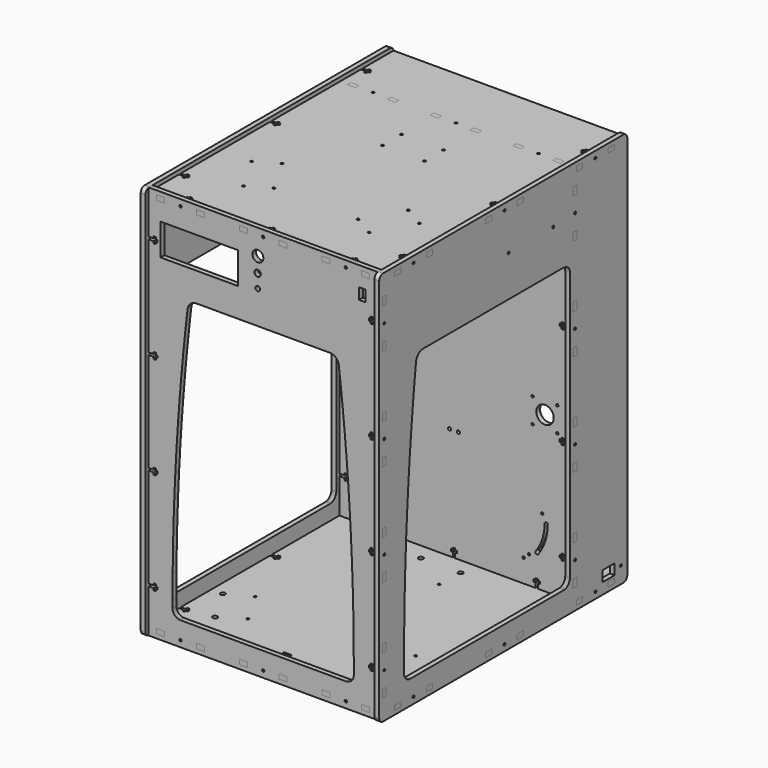
from build123d import *

# Parameters (mm, degrees)
F2_R      = 1.5
F2_W      = 10
F2_H      = 6
F3_DEPTH  = 6
F4_R      = 3
F4_R_2    = 1.5
F4_W      = 10
F4_H      = 6
F4_H_2    = 6.01
F4_W_2    = 5
F4_H_3    = 5
F5_DEPTH  = 6
F8_W      = 6
F8_H      = 10
F8_W_2    = 10
F8_H_2    = 6
F8_R      = 1.5
F8_W_3    = 19
F8_H_3    = 13.3
F9_DEPTH  = 6
F10_R     = 1.5
F11_DEPTH = 6
F13_W     = 10
F13_H     = 6
F13_W_2   = 97.175341
F13_H_2   = 39.69992
F14_DEPTH = 6
F16_R     = 1.5
F16_R_2   = 11
F16_R_3   = 2
F16_W     = 12
F16_H     = 30
F17_DEPTH = 6


# Not quite as in the source:
# - ends of sketch curves that miss each other by under 0.0002 mm in the source are joined


with BuildPart() as f3:
    # F2 (on offset) → F3 (new body)
    with BuildSketch(Plane.XY.offset(237.15)):
        Polygon((-150, 159.5), (-144, 159.5), (-144, 141), (-138, 141), (-138, 143.5), (-135, 143.5), (-135, 141), (-133, 141), (-133, 138), (-135, 138), (-135, 135.5), (-138, 135.5), (-138, 138), (-144, 138), (-144, 119.5), (-150, 119.5), (-150, 109.5), (-144, 109.5), (-144, 26.50564), (-150, 26.50564), (-150, 16.50564), (-144, 16.50564), (-144, -1.99436), (-138, -1.99436), (-138, 0.50564), (-135, 0.50564), (-135, -1.99436), (-133, -1.99436), (-133, -4.99436), (-135, -4.99436), (-135, -7.49436), (-138, -7.49436), (-138, -4.99436), (-144, -4.99436), (-144, -23.49436), (-150, -23.49436), (-150, -33.49436), (-144, -33.49436), (-144, -116.493928), (-150, -116.493928), (-150, -126.493928), (-144, -126.493928), (-144, -144.993928), (-138, -144.993928), (-138, -142.493928), (-135, -142.493928), (-135, -144.993928), (-133, -144.993928), (-133, -147.993928), (-135, -147.993928), (-135, -150.493928), (-138, -150.493928), (-138, -147.993928), (-144, -147.993928), (-144, -166.493928), (-150, -166.493928), (-150, -176.493928), (-144, -176.493928), (-144, -189.5), (-134, -189.500001), (-134, -195.500018), (-124, -195.500018), (-124, -189.500001), (-105.5, -189.500001), (-105.5, -183.5), (-108, -183.5), (-108, -180.500001), (-105.5, -180.500001), (-105.5, -178.5), (-102.5, -178.5), (-102.5, -180.500001), (-100, -180.500001), (-100, -183.5), (-102.5, -183.5), (-102.5, -189.500001), (-84, -189.500001), (-84, -195.500018), (-74, -195.500018), (-74, -189.500001), (-30, -189.5), (-30, -195.500018), (-20, -195.500018), (-20, -189.5), (-1.5, -189.5), (-1.5, -183.5), (-4, -183.5), (-4, -180.5), (-1.5, -180.5), (-1.5, -178.5), (1.5, -178.5), (1.5, -180.5), (4, -180.5), (4, -183.5), (1.5, -183.5), (1.5, -189.5), (20, -189.5), (20, -195.500018), (30, -195.500018), (30, -189.5), (74, -189.5), (74, -195.500018), (84, -195.500018), (84, -189.5), (102.5, -189.5), (102.5, -183.5), (100, -183.5), (100, -180.5), (102.5, -180.5), (102.5, -178.5), (105.5, -178.5), (105.5, -180.5), (108, -180.5), (108, -183.5), (105.5, -183.5), (105.5, -189.5), (124, -189.5), (124, -195.500018), (134, -195.500018), (134, -189.5), (144, -189.500001), (144, -176.49978), (150, -176.49978), (150, -166.49978), (144, -166.49978), (144, -147.99978), (138, -147.99978), (138, -150.49978), (135, -150.49978), (135, -147.99978), (133, -147.99978), (133, -144.99978), (135, -144.99978), (135, -142.49978), (138, -142.49978), (138, -144.99978), (144, -144.99978), (144, -126.49978), (150, -126.49978), (150, -116.49978), (144, -116.49978), (144, -33.500211), (150, -33.500211), (150, -23.500211), (144, -23.500211), (144, -5.000211), (138, -5.000211), (138, -7.500211), (135, -7.500211), (135, -5.000211), (133, -5.000211), (133, -2.000211), (135, -2.000211), (135, 0.499789), (138, 0.499789), (138, -2.000211), (144, -2.000211), (144, 16.499789), (150, 16.499789), (150, 26.499789), (144, 26.499789), (144, 109.494148), (150, 109.494148), (150, 119.494148), (144, 119.494148), (144, 137.994148), (138, 137.994148), (138, 135.494148), (135, 135.494148), (135, 137.994148), (133, 137.994148), (133, 140.994148), (135, 140.994148), (135, 143.494148), (138, 143.494148), (138, 140.994148), (144, 140.994148), (144, 159.494148), (150, 159.494148), (150, 169.494148), (144, 169.494148), (144, 189.5), (-144, 189.5), (-144, 169.5), (-150, 169.5), align=None)
        with Locations((-78.981705, -127.549038)):
            Circle(F2_R, mode=Mode.SUBTRACT)
        with Locations((-53.000943, -112.549038)):
            Circle(F2_R, mode=Mode.SUBTRACT)
        with Locations((-105.481705, -81.649692)):
            Circle(F2_R, mode=Mode.SUBTRACT)
        with Locations((-79.500943, -66.649692)):
            Circle(F2_R, mode=Mode.SUBTRACT)
        with Locations((53.000943, -112.549038)):
            Circle(F2_R, mode=Mode.SUBTRACT)
        with Locations((78.981706, -127.549038)):
            Circle(F2_R, mode=Mode.SUBTRACT)
        with Locations((105.481706, -81.649692)):
            Circle(F2_R, mode=Mode.SUBTRACT)
        with Locations((79.500943, -66.649692)):
            Circle(F2_R, mode=Mode.SUBTRACT)
        with Locations((-26.5, 25.150635)):
            Circle(F2_R, mode=Mode.SUBTRACT)
        with Locations((-26.5, 55.150635)):
            Circle(F2_R, mode=Mode.SUBTRACT)
        with Locations((-129, 107.5)):
            Rectangle(F2_W, F2_H, mode=Mode.SUBTRACT)
        with Locations((-104, 107.5)):
            Circle(F2_R, mode=Mode.SUBTRACT)
        with Locations((-79, 107.5)):
            Rectangle(F2_W, F2_H, mode=Mode.SUBTRACT)
        with Locations((-25, 107.5)):
            Rectangle(F2_W, F2_H, mode=Mode.SUBTRACT)
        with Locations((26.5, 25.150635)):
            Circle(F2_R, mode=Mode.SUBTRACT)
        with Locations((26.5, 55.150635)):
            Circle(F2_R, mode=Mode.SUBTRACT)
        with Locations((0, 107.5)):
            Circle(F2_R, mode=Mode.SUBTRACT)
        with Locations((25, 107.5)):
            Rectangle(F2_W, F2_H, mode=Mode.SUBTRACT)
        with Locations((79.000003, 107.505851)):
            Rectangle(F2_W, F2_H, mode=Mode.SUBTRACT)
        with Locations((104.000003, 107.505851)):
            Circle(F2_R, mode=Mode.SUBTRACT)
        with Locations((129.000003, 107.505851)):
            Rectangle(F2_W, F2_H, mode=Mode.SUBTRACT)
    extrude(amount=F3_DEPTH)


with BuildPart() as f5:
    # F4 (on offset) → F5 (new body)
    with BuildSketch(Plane.XY.offset(-237.15)):
        Polygon((134, -195.5000055), (134, -189.5000055), (144, -189.5000055), (144, -176.4997665), (150, -176.4997665), (150, -166.4997665), (144, -166.4997665), (144, -147.9997665), (138, -147.9997665), (138, -150.4997665), (135, -150.4997665), (135, -147.9997665), (133, -147.9997665), (133, -144.9997665), (135, -144.9997665), (135, -142.4997665), (138, -142.4997665), (138, -144.9997665), (144, -144.9997665), (144, -126.4997665), (150, -126.4997665), (150, -116.4997665), (144, -116.4997665), (144, -33.5001985), (150, -33.5001985), (150, -23.5001985), (144, -23.5001985), (144, -5.0001985), (138, -5.0001985), (138, -7.5001985), (135, -7.5001985), (135, -5.0001985), (133, -5.0001985), (133, -2.0001985), (135, -2.0001985), (135, 0.4998015), (138, 0.4998015), (138, -2.0001985), (144, -2.0001985), (144, 16.4998015), (150, 16.4998015), (150, 26.4998015), (144, 26.4998015), (144, 109.5000125), (150, 109.5000125), (150, 119.5000125), (144, 119.5000125), (144, 138.0000125), (138, 138.0000125), (138, 135.5000125), (135, 135.5000125), (135, 138.0000125), (133, 138.0000125), (133, 141.0000125), (135, 141.0000125), (135, 143.5000125), (138, 143.5000125), (138, 141.0000125), (144, 141.0000125), (144, 159.5000125), (150, 159.5000125), (150, 169.5000125), (144, 169.5000125), (144, 189.5000055), (-144, 189.5000055), (-144, 169.5000065), (-150, 169.5000065), (-150, 159.5000065), (-144, 159.5000065), (-144, 141.0000065), (-138, 141.0000065), (-138, 143.5000065), (-135, 143.5000065), (-135, 141.0000065), (-133, 141.0000065), (-133, 138.0000065), (-135, 138.0000065), (-135, 135.5000065), (-138, 135.5000065), (-138, 138.0000065), (-144, 138.0000065), (-144, 119.5000065), (-150, 119.5000065), (-150, 109.5000065), (-144, 109.5000065), (-144, 26.4998015), (-150, 26.4998015), (-150, 16.4998015), (-144, 16.4998015), (-144, -2.0001985), (-138, -2.0001985), (-138, 0.4998015), (-135, 0.4998015), (-135, -2.0001985), (-133, -2.0001985), (-133, -5.0001985), (-135, -5.0001985), (-135, -7.5001985), (-138, -7.5001985), (-138, -5.0001985), (-144, -5.0001985), (-144, -23.5001985), (-150, -23.5001985), (-150, -33.5001985), (-144, -33.5001985), (-144, -116.4997665), (-150, -116.4997665), (-150, -126.4997665), (-144, -126.4997665), (-144, -144.9997665), (-138, -144.9997665), (-138, -142.4997665), (-135, -142.4997665), (-135, -144.9997665), (-133, -144.9997665), (-133, -147.9997665), (-135, -147.9997665), (-135, -150.4997665), (-138, -150.4997665), (-138, -147.9997665), (-144, -147.9997665), (-144, -166.4997665), (-150, -166.4997665), (-150, -176.4997665), (-144, -176.4997665), (-144, -189.5000055), (-134, -189.5000055), (-134, -195.5000055), (-124, -195.5000055), (-124, -189.5000055), (-105.5, -189.5000055), (-105.5, -183.5000055), (-108, -183.5000055), (-108, -180.5000055), (-105.5, -180.5000055), (-105.5, -178.5000055), (-102.5, -178.5000055), (-102.5, -180.5000055), (-100, -180.5000055), (-100, -183.5000055), (-102.5, -183.5000055), (-102.5, -189.5000055), (-84, -189.5000055), (-84, -195.5000055), (-74, -195.5000055), (-74, -189.5000055), (-30, -189.5000055), (-30, -195.5000055), (-20, -195.5000055), (-20, -189.5000055), (-1.5, -189.5000055), (-1.5, -183.5000055), (-4, -183.5000055), (-4, -180.5000055), (-1.5, -180.5000055), (-1.5, -178.5000055), (1.5, -178.5000055), (1.5, -180.5000055), (4, -180.5000055), (4, -183.5000055), (1.5, -183.5000055), (1.5, -189.5000055), (20, -189.5000055), (20, -195.5000055), (30, -195.5000055), (30, -189.5000055), (74, -189.5000055), (74, -195.5000055), (84, -195.5000055), (84, -189.5000055), (102.5, -189.5000055), (102.5, -183.5000055), (100, -183.5000055), (100, -180.5000055), (102.5, -180.5000055), (102.5, -178.5000055), (105.5, -178.5000055), (105.5, -180.5000055), (108, -180.5000055), (108, -183.5000055), (105.5, -183.5000055), (105.5, -189.5000055), (124, -189.5000055), (124, -195.5000055), align=None)
        with Locations((-104.41343, -140.5001355)):
            Circle(F4_R, mode=Mode.SUBTRACT)
        with Locations((-76.946027, -123.4871225)):
            Circle(F4_R_2, mode=Mode.SUBTRACT)
        with BuildLine():
            ThreePointArc((-3.529365, -159.5495045), (-5.029365, -158.0495045), (-3.529365, -156.5495045))
            Line((-3.529365, -156.5495045), (3.470635, -156.5495045))
            ThreePointArc((3.470635, -156.5495045), (4.970635, -158.0495045), (3.470635, -159.5495045))
            Line((3.470635, -159.5495045), (-3.529365, -159.5495045))
        make_face(mode=Mode.SUBTRACT)
        with Locations((-129.41343, -97.1988655)):
            Circle(F4_R, mode=Mode.SUBTRACT)
        with Locations((-100.946027, -81.9179035)):
            Circle(F4_R_2, mode=Mode.SUBTRACT)
        with Locations((76.946027, -123.4871225)):
            Circle(F4_R_2, mode=Mode.SUBTRACT)
        with Locations((104.41343, -140.5001355)):
            Circle(F4_R, mode=Mode.SUBTRACT)
        with Locations((100.946027, -81.9179035)):
            Circle(F4_R_2, mode=Mode.SUBTRACT)
        with Locations((129.41343, -97.1988655)):
            Circle(F4_R, mode=Mode.SUBTRACT)
        with Locations((-24, 51.3565255)):
            Circle(F4_R_2, mode=Mode.SUBTRACT)
        with Locations((-25, 83.6504995)):
            Circle(F4_R, mode=Mode.SUBTRACT)
        with Locations((-129, 107.4998645)):
            Rectangle(F4_W, F4_H, mode=Mode.SUBTRACT)
        with Locations((-104, 107.4998645)):
            Circle(F4_R_2, mode=Mode.SUBTRACT)
        with Locations((-79, 107.4998645)):
            Rectangle(F4_W, F4_H, mode=Mode.SUBTRACT)
        with Locations((-25, 107.4998645)):
            Rectangle(F4_W, F4_H, mode=Mode.SUBTRACT)
        with Locations((24, 51.3565255)):
            Circle(F4_R_2, mode=Mode.SUBTRACT)
        with Locations((25, 83.6504995)):
            Circle(F4_R, mode=Mode.SUBTRACT)
        with Locations((0, 107.4998645)):
            Circle(F4_R_2, mode=Mode.SUBTRACT)
        with Locations((25, 107.4998645)):
            Rectangle(F4_W, F4_H, mode=Mode.SUBTRACT)
        with Locations((79, 107.4998645)):
            Rectangle(F4_W, F4_H, mode=Mode.SUBTRACT)
        with Locations((104, 107.4998645)):
            Circle(F4_R_2, mode=Mode.SUBTRACT)
        with Locations((129, 107.5048645)):
            Rectangle(F4_W, F4_H_2, mode=Mode.SUBTRACT)
        with Locations((136.5, 117.9998645)):
            Rectangle(F4_W_2, F4_H_3, mode=Mode.SUBTRACT)
    extrude(amount=-F5_DEPTH)


with BuildPart() as f9:
    # F8 (on offset) → F9 (new body)
    with BuildSketch(Plane.YZ.offset(144)):
        with BuildLine():
            Line((189.499992, -242.15), (189.499402, 242.149892))
            Line((189.499402, 242.149892), (189.294966, 243.702831))
            Line((189.294966, 243.702831), (188.695564, 245.149942))
            Line((188.695564, 245.149942), (187.742044, 246.392606))
            Line((187.742044, 246.392606), (186.499388, 247.346136))
            Line((186.499388, 247.346136), (185.052282, 247.945551))
            Line((185.052282, 247.945551), (183.499344, 248.15))
            Line((183.499344, 248.15), (-194.499763, 248.15))
            ThreePointArc((-194.499763, 248.15), (-198.7423994455, 246.3927505531), (-200.499779, 242.150168))
            Line((-200.499779, 242.150168), (-200.499888, -242.15))
            Line((-200.499888, -242.15), (-200.295444, -243.702914))
            Line((-200.295444, -243.702914), (-199.696041, -245.15))
            Line((-199.696041, -245.15), (-198.74253, -246.392641))
            Line((-198.74253, -246.392641), (-197.499889, -247.346152))
            Line((-197.499889, -247.346152), (-196.052804, -247.945555))
            Line((-196.052804, -247.945555), (-194.49989, -248.15))
            Line((-194.49989, -248.15), (183.5, -248.15))
            ThreePointArc((183.5, -248.15), (187.7426382122, -246.3926402625), (189.499992, -242.15))
        make_face()
        with Locations((-192.500018, -217.15)):
            Rectangle(F8_W, F8_H, mode=Mode.SUBTRACT)
        with Locations((-171.49978, -240.15)):
            Rectangle(F8_W_2, F8_H_2, mode=Mode.SUBTRACT)
        with Locations((-192.500018, -192.15)):
            Circle(F8_R, mode=Mode.SUBTRACT)
        Polygon((-144.99978, -240.15), (-145.050891, -240.538229), (-145.200742, -240.9), (-145.43912, -241.21066), (-145.74978, -241.449038), (-146.111552, -241.598889), (-146.49978, -241.65), (-146.888009, -241.598889), (-147.24978, -241.449038), (-147.56044, -241.21066), (-147.798818, -240.9), (-147.948669, -240.538229), (-147.99978, -240.15), (-147.948669, -239.761771), (-147.798818, -239.4), (-147.56044, -239.08934), (-147.24978, -238.850962), (-146.888009, -238.701111), (-146.49978, -238.65), (-146.111552, -238.701111), (-145.74978, -238.850962), (-145.43912, -239.08934), (-145.200742, -239.4), (-145.050891, -239.761771), align=None, mode=Mode.SUBTRACT)
        with Locations((-121.49978, -240.15)):
            Rectangle(F8_W_2, F8_H_2, mode=Mode.SUBTRACT)
        with Locations((-192.500018, -167.15)):
            Rectangle(F8_W, F8_H, mode=Mode.SUBTRACT)
        with Locations((-28.500211, -240.15)):
            Rectangle(F8_W_2, F8_H_2, mode=Mode.SUBTRACT)
        with Locations((-192.500018, -89.05)):
            Rectangle(F8_W, F8_H, mode=Mode.SUBTRACT)
        Polygon((-191.05113, -63.661771), (-191.000018, -64.05), (-191.05113, -64.438229), (-191.20098, -64.8), (-191.439358, -65.11066), (-191.750018, -65.349038), (-192.11179, -65.498889), (-192.500018, -65.55), (-192.888247, -65.498889), (-193.250018, -65.349038), (-193.560679, -65.11066), (-193.799056, -64.8), (-193.948907, -64.438229), (-194.000018, -64.05), (-193.948907, -63.661771), (-193.799056, -63.3), (-193.560679, -62.98934), (-193.250018, -62.750962), (-192.888247, -62.601111), (-192.500018, -62.55), (-192.11179, -62.601111), (-191.750018, -62.750962), (-191.439358, -62.98934), (-191.20098, -63.3), align=None, mode=Mode.SUBTRACT)
        with Locations((-192.500018, -39.05)):
            Rectangle(F8_W, F8_H, mode=Mode.SUBTRACT)
        with BuildLine():
            Line((90.805261, -218.064449), (89.5, -218.15))
            Line((89.5, -218.15), (-151.499902, -218.15))
            Line((-151.499902, -218.15), (-152.805163, -218.064449))
            Line((-152.805163, -218.064449), (-154.088092, -217.809258))
            Line((-154.088092, -217.809258), (-155.326736, -217.388795))
            Line((-155.326736, -217.388795), (-156.499902, -216.810254))
            Line((-156.499902, -216.810254), (-157.587516, -216.083533))
            Line((-157.587516, -216.083533), (-158.570969, -215.221068))
            Line((-158.570969, -215.221068), (-159.433435, -214.237614))
            Line((-159.433435, -214.237614), (-160.160156, -213.15))
            Line((-160.160156, -213.15), (-160.738697, -211.976834))
            Line((-160.738697, -211.976834), (-161.15916, -210.73819))
            Line((-161.15916, -210.73819), (-161.41435, -209.455262))
            Line((-161.41435, -209.455262), (-161.499902, -208.15))
            Line((-161.499902, -208.15), (-161.499904, -198.15))
            Line((-161.499904, -198.15), (-161.360861, -169.976288))
            Line((-161.360861, -169.976288), (-160.943732, -141.805321))
            Line((-160.943732, -141.805321), (-160.248556, -113.639844))
            Line((-160.248556, -113.639844), (-159.275401, -85.482601))
            Line((-159.275401, -85.482601), (-158.024363, -57.336335))
            Line((-158.024363, -57.336335), (-156.495562, -29.203789))
            Line((-156.495562, -29.203789), (-154.689149, -1.087704))
            Line((-154.689149, -1.087704), (-152.605299, 27.00918))
            Line((-152.605299, 27.00918), (-150.244215, 55.084128))
            Line((-150.244215, 55.084128), (-147.606127, 83.134401))
            Line((-147.606127, 83.134401), (-144.691292, 111.157269))
            Line((-144.691292, 111.157269), (-142.64004, 129.15))
            Line((-142.64004, 129.15), (-142.402772, 130.497965))
            Line((-142.402772, 130.497965), (-142.003956, 131.80726))
            Line((-142.003956, 131.80726), (-141.449468, 133.058599))
            Line((-141.449468, 133.058599), (-140.747473, 134.23355))
            Line((-140.747473, 134.23355), (-139.908313, 135.314807))
            Line((-139.908313, 135.314807), (-138.944347, 136.286443))
            Line((-138.944347, 136.286443), (-137.869775, 137.134146))
            Line((-137.869775, 137.134146), (-136.700425, 137.845431))
            Line((-136.700425, 137.845431), (-135.45352, 138.40982))
            Line((-135.45352, 138.40982), (-134.147427, 138.819))
            Line((-134.147427, 138.819), (-132.801385, 139.066944))
            Line((-132.801385, 139.066944), (-131.435219, 139.15))
            Line((-131.435219, 139.15), (89.5, 139.15))
            ThreePointArc((89.5, 139.15), (96.5710678119, 136.2210678119), (99.5, 129.15))
            Line((99.5, 129.15), (99.5, -208.15))
            Line((99.5, -208.15), (99.414448, -209.455262))
            Line((99.414448, -209.455262), (99.159258, -210.73819))
            Line((99.159258, -210.73819), (98.738795, -211.976834))
            Line((98.738795, -211.976834), (98.160254, -213.15))
            Line((98.160254, -213.15), (97.433533, -214.237614))
            Line((97.433533, -214.237614), (96.571067, -215.221068))
            Line((96.571067, -215.221068), (95.587614, -216.083533))
            Line((95.587614, -216.083533), (94.5, -216.810254))
            Line((94.5, -216.810254), (93.326834, -217.388795))
            Line((93.326834, -217.388795), (92.08819, -217.809258))
            Line((92.08819, -217.809258), (90.805261, -218.064449))
        make_face(mode=Mode.SUBTRACT)
        Polygon((-2.439551, -239.08934), (-2.201173, -239.4), (-2.051323, -239.761771), (-2.000211, -240.15), (-2.051323, -240.538229), (-2.201173, -240.9), (-2.439551, -241.21066), (-2.750211, -241.449038), (-3.111983, -241.598889), (-3.500211, -241.65), (-3.88844, -241.598889), (-4.250211, -241.449038), (-4.560872, -241.21066), (-4.799249, -240.9), (-4.9491, -240.538229), (-5.000211, -240.15), (-4.9491, -239.761771), (-4.799249, -239.4), (-4.560872, -239.08934), (-4.250211, -238.850962), (-3.88844, -238.701111), (-3.500211, -238.65), (-3.111983, -238.701111), (-2.750211, -238.850962), align=None, mode=Mode.SUBTRACT)
        with Locations((21.499789, -240.15)):
            Rectangle(F8_W_2, F8_H_2, mode=Mode.SUBTRACT)
        with Locations((114.5, -240.15)):
            Rectangle(F8_W_2, F8_H_2, mode=Mode.SUBTRACT)
        with Locations((107.505851, -217.15)):
            Rectangle(F8_W, F8_H, mode=Mode.SUBTRACT)
        Polygon((140.56066, -239.08934), (140.799038, -239.4), (140.948888, -239.761771), (141, -240.15), (140.948888, -240.538229), (140.799038, -240.9), (140.56066, -241.21066), (140.25, -241.449038), (139.888228, -241.598889), (139.5, -241.65), (139.111771, -241.598889), (138.75, -241.449038), (138.439339, -241.21066), (138.200961, -240.9), (138.051111, -240.538229), (138, -240.15), (138.051111, -239.761771), (138.200961, -239.4), (138.439339, -239.08934), (138.75, -238.850962), (139.111771, -238.701111), (139.5, -238.65), (139.888228, -238.701111), (140.25, -238.850962), align=None, mode=Mode.SUBTRACT)
        Polygon((106.056963, -191.761771), (106.206813, -191.4), (106.445191, -191.08934), (106.755851, -190.850962), (107.117623, -190.701111), (107.505851, -190.65), (107.89408, -190.701111), (108.255851, -190.850962), (108.566511, -191.08934), (108.804889, -191.4), (108.95474, -191.761771), (109.005851, -192.15), (108.95474, -192.538229), (108.804889, -192.9), (108.566511, -193.21066), (108.255851, -193.449038), (107.89408, -193.598889), (107.505851, -193.65), (107.117623, -193.598889), (106.755851, -193.449038), (106.445191, -193.21066), (106.206813, -192.9), (106.056963, -192.538229), (106.005851, -192.15), align=None, mode=Mode.SUBTRACT)
        with Locations((164.5, -240.15)):
            Rectangle(F8_W_2, F8_H_2, mode=Mode.SUBTRACT)
        with Locations((160.1, -227.5)):
            Rectangle(F8_W_3, F8_H_3, mode=Mode.SUBTRACT)
        with Locations((179.500025, -227.500622)):
            Circle(F8_R, mode=Mode.SUBTRACT)
        with Locations((107.505851, -167.15)):
            Rectangle(F8_W, F8_H, mode=Mode.SUBTRACT)
        with Locations((107.505851, -89.05)):
            Rectangle(F8_W, F8_H, mode=Mode.SUBTRACT)
        Polygon((107.505851, -62.55), (107.89408, -62.601111), (108.255851, -62.750962), (108.566511, -62.98934), (108.804889, -63.3), (108.95474, -63.661771), (109.005851, -64.05), (108.95474, -64.438229), (108.804889, -64.8), (108.566511, -65.11066), (108.255851, -65.349038), (107.89408, -65.498889), (107.505851, -65.55), (107.117623, -65.498889), (106.755851, -65.349038), (106.445191, -65.11066), (106.206813, -64.8), (106.056963, -64.438229), (106.005851, -64.05), (106.056963, -63.661771), (106.206813, -63.3), (106.445191, -62.98934), (106.755851, -62.750962), (107.117623, -62.601111), align=None, mode=Mode.SUBTRACT)
        with Locations((107.505851, -39.05)):
            Rectangle(F8_W, F8_H, mode=Mode.SUBTRACT)
        with Locations((-192.500018, 39.05)):
            Rectangle(F8_W, F8_H, mode=Mode.SUBTRACT)
        Polygon((-192.11179, 62.601111), (-192.500018, 62.55), (-192.888247, 62.601111), (-193.250018, 62.750962), (-193.560679, 62.98934), (-193.799056, 63.3), (-193.948907, 63.661771), (-194.000018, 64.05), (-193.948907, 64.438229), (-193.799056, 64.8), (-193.560679, 65.11066), (-193.250018, 65.349038), (-192.888247, 65.498889), (-192.500018, 65.55), (-192.11179, 65.498889), (-191.750018, 65.349038), (-191.439358, 65.11066), (-191.20098, 64.8), (-191.05113, 64.438229), (-191.000018, 64.05), (-191.05113, 63.661771), (-191.20098, 63.3), (-191.439358, 62.98934), (-191.750018, 62.750962), align=None, mode=Mode.SUBTRACT)
        with Locations((-192.500018, 89.05)):
            Rectangle(F8_W, F8_H, mode=Mode.SUBTRACT)
        with Locations((-192.500018, 167.15)):
            Rectangle(F8_W, F8_H, mode=Mode.SUBTRACT)
        Polygon((-192.888247, 190.701111), (-193.250018, 190.850962), (-193.560679, 191.08934), (-193.799056, 191.4), (-193.948907, 191.761771), (-194.000018, 192.15), (-193.948907, 192.538229), (-193.799056, 192.9), (-193.560679, 193.21066), (-193.250018, 193.449038), (-192.888247, 193.598889), (-192.500018, 193.65), (-192.11179, 193.598889), (-191.750018, 193.449038), (-191.439358, 193.21066), (-191.20098, 192.9), (-191.05113, 192.538229), (-191.000018, 192.15), (-191.05113, 191.761771), (-191.20098, 191.4), (-191.439358, 191.08934), (-191.750018, 190.850962), (-192.11179, 190.701111), (-192.500018, 190.65), align=None, mode=Mode.SUBTRACT)
        with Locations((-192.500018, 217.15)):
            Rectangle(F8_W, F8_H, mode=Mode.SUBTRACT)
        with Locations((-171.49978, 240.15)):
            Rectangle(F8_W_2, F8_H_2, mode=Mode.SUBTRACT)
        Polygon((-145.050891, 240.538229), (-144.99978, 240.15), (-145.050891, 239.761771), (-145.200742, 239.4), (-145.43912, 239.08934), (-145.74978, 238.850962), (-146.111552, 238.701111), (-146.49978, 238.65), (-146.888009, 238.701111), (-147.24978, 238.850962), (-147.56044, 239.08934), (-147.798818, 239.4), (-147.948669, 239.761771), (-147.99978, 240.15), (-147.948669, 240.538229), (-147.798818, 240.9), (-147.56044, 241.21066), (-147.24978, 241.449038), (-146.888009, 241.598889), (-146.49978, 241.65), (-146.111552, 241.598889), (-145.74978, 241.449038), (-145.43912, 241.21066), (-145.200742, 240.9), align=None, mode=Mode.SUBTRACT)
        with Locations((-121.49978, 240.15)):
            Rectangle(F8_W_2, F8_H_2, mode=Mode.SUBTRACT)
        with Locations((-28.500211, 240.15)):
            Rectangle(F8_W_2, F8_H_2, mode=Mode.SUBTRACT)
        with Locations((107.505851, 39.05)):
            Rectangle(F8_W, F8_H, mode=Mode.SUBTRACT)
        with Locations((107.505851, 64.05)):
            Circle(F8_R, mode=Mode.SUBTRACT)
        with Locations((107.505851, 89.05)):
            Rectangle(F8_W, F8_H, mode=Mode.SUBTRACT)
        with Locations((3.031226, 190.6)):
            Circle(F8_R, mode=Mode.SUBTRACT)
        Polygon((-2.051323, 239.761771), (-2.201173, 239.4), (-2.439551, 239.08934), (-2.750211, 238.850962), (-3.111983, 238.701111), (-3.500211, 238.65), (-3.88844, 238.701111), (-4.250211, 238.850962), (-4.560872, 239.08934), (-4.799249, 239.4), (-4.9491, 239.761771), (-5.000211, 240.15), (-4.9491, 240.538229), (-4.799249, 240.9), (-4.560872, 241.21066), (-4.250211, 241.449038), (-3.88844, 241.598889), (-3.500211, 241.65), (-3.111983, 241.598889), (-2.750211, 241.449038), (-2.439551, 241.21066), (-2.201173, 240.9), (-2.051323, 240.538229), (-2.000211, 240.15), align=None, mode=Mode.SUBTRACT)
        with Locations((21.499789, 240.15)):
            Rectangle(F8_W_2, F8_H_2, mode=Mode.SUBTRACT)
        Polygon((71.582337, 190.988229), (71.732188, 191.35), (71.970566, 191.66066), (72.281226, 191.899038), (72.642998, 192.048889), (73.031226, 192.1), (73.419455, 192.048889), (73.781226, 191.899038), (74.091886, 191.66066), (74.330264, 191.35), (74.480115, 190.988229), (74.531226, 190.6), (74.480115, 190.211771), (74.330264, 189.85), (74.091886, 189.53934), (73.781226, 189.300962), (73.419455, 189.151111), (73.031226, 189.1), (72.642998, 189.151111), (72.281226, 189.300962), (71.970566, 189.53934), (71.732188, 189.85), (71.582337, 190.211771), (71.531226, 190.6), align=None, mode=Mode.SUBTRACT)
        with Locations((107.5, 167.15)):
            Rectangle(F8_W, F8_H, mode=Mode.SUBTRACT)
        Polygon((106.200961, 192.9), (106.439339, 193.21066), (106.75, 193.449038), (107.111771, 193.598889), (107.5, 193.65), (107.888228, 193.598889), (108.25, 193.449038), (108.56066, 193.21066), (108.799038, 192.9), (108.948888, 192.538229), (109, 192.15), (108.948888, 191.761771), (108.799038, 191.4), (108.56066, 191.08934), (108.25, 190.850962), (107.888228, 190.701111), (107.5, 190.65), (107.111771, 190.701111), (106.75, 190.850962), (106.439339, 191.08934), (106.200961, 191.4), (106.051111, 191.761771), (106, 192.15), (106.051111, 192.538229), align=None, mode=Mode.SUBTRACT)
        with Locations((107.5, 217.15)):
            Rectangle(F8_W, F8_H, mode=Mode.SUBTRACT)
        with Locations((114.494148, 240.15)):
            Rectangle(F8_W_2, F8_H_2, mode=Mode.SUBTRACT)
        Polygon((139.105919, 241.598889), (139.494148, 241.65), (139.882376, 241.598889), (140.244148, 241.449038), (140.554808, 241.21066), (140.793186, 240.9), (140.943037, 240.538229), (140.994148, 240.15), (140.943037, 239.761771), (140.793186, 239.4), (140.554808, 239.08934), (140.244148, 238.850962), (139.882376, 238.701111), (139.494148, 238.65), (139.105919, 238.701111), (138.744148, 238.850962), (138.433488, 239.08934), (138.19511, 239.4), (138.045259, 239.761771), (137.994148, 240.15), (138.045259, 240.538229), (138.19511, 240.9), (138.433488, 241.21066), (138.744148, 241.449038), align=None, mode=Mode.SUBTRACT)
        with Locations((164.494148, 240.15)):
            Rectangle(F8_W_2, F8_H_2, mode=Mode.SUBTRACT)
    extrude(amount=F9_DEPTH)


with BuildPart() as f11:
    # F10 (on offset) → F11 (new body)
    with BuildSketch(Plane(origin=(-144, 0, 0), x_dir=(0, -1, 0), z_dir=(-1, 0, 0))):
        with BuildLine():
            Line((-189.4994047464, 242.1501386605), (-189.5003987455, -242.1498613388))
            Line((-189.5003987455, -242.1498613388), (-189.2959570666, -243.7027755127))
            Line((-189.2959570666, -243.7027755127), (-188.6965572976, -245.1498610227))
            Line((-188.6965572976, -245.1498610227), (-187.7430483547, -246.3925028338))
            Line((-187.7430483547, -246.3925028338), (-186.5004091659, -247.3460158909))
            Line((-186.5004091659, -247.3460158909), (-185.0533246758, -247.945420122))
            Line((-185.0533246758, -247.945420122), (-183.5004118497, -248.1498664431))
            Line((-183.5004118497, -248.1498664431), (194.5006771501, -248.1501880126))
            ThreePointArc((194.5006771501, -248.1501880126), (198.7425492927, -246.393151269), (200.4995932535, -242.1512821159))
            Line((200.4995932535, -242.1512821159), (200.4997992534, 242.1497908841))
            ThreePointArc((200.4997992534, 242.1497908841), (198.7424291669, 246.3924452898), (194.4997733577, 248.1498119884))
            Line((194.4997733577, 248.1498119884), (-183.4993926421, 248.1501335562))
            ThreePointArc((-183.4993926421, 248.1501335562), (-187.7420372991, 246.3927782772), (-189.4994047464, 242.1501386605))
        make_face()
        Polygon((-159.5004015962, -243.1498868601), (-169.5004015962, -243.149878353), (-169.5003964919, -237.149878353), (-159.5003964919, -237.1498868601), align=None, mode=Mode.SUBTRACT)
        with Locations((-139.5003990441, -240.1499038743)):
            Circle(F10_R, mode=Mode.SUBTRACT)
        Polygon((-109.5004015962, -243.1499293957), (-119.5004015962, -243.1499208886), (-119.5003964919, -237.1499208886), (-109.500396492, -237.1499293957), align=None, mode=Mode.SUBTRACT)
        Polygon((-104.5062417313, -222.1499336442), (-110.5062417313, -222.14992854), (-110.5062332242, -212.14992854), (-104.5062332242, -212.1499336442), align=None, mode=Mode.SUBTRACT)
        with Locations((-107.50621621, -192.1499310921)):
            Circle(F10_R, mode=Mode.SUBTRACT)
        Polygon((-104.5061991958, -172.1499336443), (-110.5061991958, -172.14992854), (-110.5061906887, -162.14992854), (-104.5061906887, -162.1499336443), align=None, mode=Mode.SUBTRACT)
        Polygon((-16.506043492, -237.1500085069), (-16.5060485962, -243.1500085069), (-26.5060485962, -243.1499999998), (-26.506043492, -237.1499999998), align=None, mode=Mode.SUBTRACT)
        Polygon((2.0450656256, -240.5382532886), (1.9939539559, -240.1500242451), (2.0450662861, -239.7617952886), (2.1949165939, -239.400024416), (2.4332948582, -239.0893646188), (2.743955061, -238.8509868831), (3.1057271885, -238.7011361909), (3.4939552319, -238.6500255211), (3.8821841885, -238.7011368514), (4.243955061, -238.8509881592), (4.5546158582, -239.0893664235), (4.7929925939, -239.4000266262), (4.9428432861, -239.7617977537), (4.9939539559, -240.1500267972), (4.9428426256, -240.5382557537), (4.7929913178, -240.9000266262), (4.5546140536, -241.2106864235), (4.2439528508, -241.4490641592), (3.8821817233, -241.5989148514), (3.4939526798, -241.6500255211), (3.1057247233, -241.5989141909), (2.7439528508, -241.4490628831), (2.4332930536, -241.2106846188), (2.1949153178, -240.900024416), align=None, mode=Mode.SUBTRACT)
        Polygon((-110.5061242482, -84.04992854), (-104.5061242482, -84.0499336443), (-104.5061327553, -94.0499336443), (-110.5061327553, -94.04992854), align=None, mode=Mode.SUBTRACT)
        Polygon((-107.50610851, -65.5499310922), (-107.8943364666, -65.4988197619), (-108.2561083391, -65.3489684541), (-108.5667681363, -65.1105901898), (-108.805145872, -64.7999299871), (-108.9549955642, -64.4381588596), (-109.006107234, -64.0499298161), (-108.9549949037, -63.6617008596), (-108.8051445959, -63.2999299871), (-108.5667663317, -62.9892701898), (-108.2561061289, -62.7508924541), (-107.8943340014, -62.6010417619), (-107.5061059579, -62.5499310922), (-107.1178770014, -62.6010424224), (-106.7561061289, -62.7508937302), (-106.4454453317, -62.9892719945), (-106.2070675959, -63.2999321973), (-106.0572179037, -63.6617033247), (-106.006107234, -64.0499323682), (-106.0572185642, -64.4381613247), (-106.207068872, -64.7999321973), (-106.4454471363, -65.1105919945), (-106.7561083391, -65.3489697302), (-107.1178794666, -65.4988204224), align=None, mode=Mode.SUBTRACT)
        Polygon((-104.5060902198, -44.0499336443), (-110.5060902198, -44.04992854), (-110.5060817127, -34.04992854), (-104.5060817127, -34.0499336443), align=None, mode=Mode.SUBTRACT)
        Polygon((33.4939514037, -243.1500510425), (23.4939514037, -243.1500425354), (23.493956508, -237.1500425354), (33.493956508, -237.1500510425), align=None, mode=Mode.SUBTRACT)
        Polygon((126.493525508, -237.1501301582), (126.4935204037, -243.1501301582), (116.4935204037, -243.1501216511), (116.493525508, -237.1501216511), align=None, mode=Mode.SUBTRACT)
        with Locations((146.4935229558, -240.1501471724)):
            Circle(F10_R, mode=Mode.SUBTRACT)
        Polygon((166.4935204037, -243.1501641866), (166.4935255079, -237.1501641866), (176.4935255079, -237.1501726937), (176.4935204037, -243.1501726937), align=None, mode=Mode.SUBTRACT)
        Polygon((189.4996282686, -222.1501837581), (189.4996367757, -212.1501837581), (195.4996367757, -212.1501888624), (195.4996282686, -222.1501888624), align=None, mode=Mode.SUBTRACT)
        with Locations((192.4996537899, -192.1501863103)):
            Circle(F10_R, mode=Mode.SUBTRACT)
        Polygon((195.4996793112, -162.1501888624), (195.4996708041, -172.1501888624), (189.4996708041, -172.1501837581), (189.4996793112, -162.1501837581), align=None, mode=Mode.SUBTRACT)
        with BuildLine():
            Line((159.4333047563, -214.2375476443), (158.5708387563, -215.2210016443))
            Line((158.5708387563, -215.2210016443), (157.5873857563, -216.0834666443))
            Line((157.5873857563, -216.0834666443), (156.4997717563, -216.8101876443))
            Line((156.4997717563, -216.8101876443), (155.3266057563, -217.3887286443))
            Line((155.3266057563, -217.3887286443), (154.0879617563, -217.8091916443))
            Line((154.0879617563, -217.8091916443), (152.8050327563, -218.0643826443))
            Line((152.8050327563, -218.0643826443), (151.4997717563, -218.1499336443))
            Line((151.4997717563, -218.1499336443), (-89.5001302437, -218.1499336443))
            Line((-89.5001302437, -218.1499336443), (-90.8053912437, -218.0643826443))
            Line((-90.8053912437, -218.0643826443), (-92.0883202437, -217.8091916443))
            Line((-92.0883202437, -217.8091916443), (-93.3269642437, -217.3887286443))
            Line((-93.3269642437, -217.3887286443), (-94.5001302437, -216.8101876443))
            Line((-94.5001302437, -216.8101876443), (-95.5877442437, -216.0834666443))
            Line((-95.5877442437, -216.0834666443), (-96.5711972437, -215.2210016443))
            Line((-96.5711972437, -215.2210016443), (-97.4336632437, -214.2375476443))
            Line((-97.4336632437, -214.2375476443), (-98.1603842437, -213.1499336443))
            Line((-98.1603842437, -213.1499336443), (-98.7389252437, -211.9767676443))
            Line((-98.7389252437, -211.9767676443), (-99.1593882437, -210.7381236443))
            Line((-99.1593882437, -210.7381236443), (-99.4145782437, -209.4551956443))
            Line((-99.4145782437, -209.4551956443), (-99.5001302437, -208.1499336443))
            Line((-99.5001302437, -208.1499336443), (-99.5001302437, 129.1500663557))
            ThreePointArc((-99.5001302437, 129.1500663557), (-96.5711980556, 136.2211341675), (-89.5001302437, 139.1500663557))
            Line((-89.5001302437, 139.1500663557), (131.4350887563, 139.1500663557))
            Line((131.4350887563, 139.1500663557), (132.8012547563, 139.0670103557))
            Line((132.8012547563, 139.0670103557), (134.1472967563, 138.8190663557))
            Line((134.1472967563, 138.8190663557), (135.4533897563, 138.4098863557))
            Line((135.4533897563, 138.4098863557), (136.7002947563, 137.8454973557))
            Line((136.7002947563, 137.8454973557), (137.8696447563, 137.1342123557))
            Line((137.8696447563, 137.1342123557), (138.9442167563, 136.2865093557))
            Line((138.9442167563, 136.2865093557), (139.9081827563, 135.3148733557))
            Line((139.9081827563, 135.3148733557), (140.7473427563, 134.2336163557))
            Line((140.7473427563, 134.2336163557), (141.4493377563, 133.0586653557))
            Line((141.4493377563, 133.0586653557), (142.0038257563, 131.8073263557))
            Line((142.0038257563, 131.8073263557), (142.4026417563, 130.4980313557))
            Line((142.4026417563, 130.4980313557), (142.6399097563, 129.1500663557))
            Line((142.6399097563, 129.1500663557), (144.6911617563, 111.1573353557))
            Line((144.6911617563, 111.1573353557), (147.6059967563, 83.1344673557))
            Line((147.6059967563, 83.1344673557), (150.2440847563, 55.0841943557))
            Line((150.2440847563, 55.0841943557), (152.6051687563, 27.0092463557))
            Line((152.6051687563, 27.0092463557), (154.6890187563, -1.0876376443))
            Line((154.6890187563, -1.0876376443), (156.4954317563, -29.2037226443))
            Line((156.4954317563, -29.2037226443), (158.0242327563, -57.3362686443))
            Line((158.0242327563, -57.3362686443), (159.2752707563, -85.4825346443))
            Line((159.2752707563, -85.4825346443), (160.2484257563, -113.6397776443))
            Line((160.2484257563, -113.6397776443), (160.9436017563, -141.8052546443))
            Line((160.9436017563, -141.8052546443), (161.3607307563, -169.9762216443))
            Line((161.3607307563, -169.9762216443), (161.4997737563, -198.1499336443))
            Line((161.4997737563, -198.1499336443), (161.4997717563, -208.1499336443))
            Line((161.4997717563, -208.1499336443), (161.4142197563, -209.4551956443))
            Line((161.4142197563, -209.4551956443), (161.1590297563, -210.7381236443))
            Line((161.1590297563, -210.7381236443), (160.7385667563, -211.9767676443))
            Line((160.7385667563, -211.9767676443), (160.1600257563, -213.1499336443))
            Line((160.1600257563, -213.1499336443), (159.4333047563, -214.2375476443))
        make_face(mode=Mode.SUBTRACT)
        Polygon((189.4997457517, -84.0501837582), (195.4997457517, -84.0501888624), (195.4997372446, -94.0501888624), (189.4997372446, -94.0501837582), align=None, mode=Mode.SUBTRACT)
        with Locations((192.4997627659, -64.0501863103)):
            Circle(F10_R, mode=Mode.SUBTRACT)
        Polygon((189.4997882872, -34.0501837582), (195.4997882872, -34.0501888624), (195.4997797801, -44.0501888624), (189.4997797801, -44.0501837582), align=None, mode=Mode.SUBTRACT)
        Polygon((-110.5060152722, 44.0500714599), (-104.5060152722, 44.0500663557), (-104.5060237793, 34.0500663557), (-110.5060237793, 34.0500714599), align=None, mode=Mode.SUBTRACT)
        Polygon((-106.206959896, 63.3000678027), (-106.4453381603, 62.9894080055), (-106.7559993631, 62.7510302698), (-107.1177704905, 62.6011795775), (-107.505999534, 62.5500689078), (-107.8942274905, 62.6011802381), (-108.2559993631, 62.7510315458), (-108.5666591603, 62.9894098101), (-108.805036896, 63.3000700129), (-108.9548865882, 63.6618411404), (-109.005998258, 64.0500701839), (-108.9548859277, 64.4382991404), (-108.8050356199, 64.8000700129), (-108.5666573556, 65.1107298101), (-108.2559971528, 65.3491075458), (-107.8942250254, 65.4989582381), (-107.5059969819, 65.5500689078), (-107.1177680254, 65.4989575775), (-106.7559971529, 65.3491062698), (-106.4453363556, 65.1107280055), (-106.2069586199, 64.8000678027), (-106.0571089277, 64.4382966752), (-106.005998258, 64.0500676317), (-106.0571095882, 63.6618386752), align=None, mode=Mode.SUBTRACT)
        Polygon((-104.5059812437, 84.0500663557), (-110.5059812437, 84.0500714599), (-110.5059727366, 94.0500714599), (-104.5059727366, 94.0500663556), align=None, mode=Mode.SUBTRACT)
        Polygon((-104.5000628033, 162.1500663506), (-110.5000628033, 162.1500714549), (-110.5000542962, 172.1500714549), (-104.5000542962, 172.1500663506), align=None, mode=Mode.SUBTRACT)
        Polygon((-159.4999938957, 243.1501131397), (-159.499999, 237.1501131397), (-169.499999, 237.1501216468), (-169.4999938957, 243.1501216468), align=None, mode=Mode.SUBTRACT)
        with Locations((-107.5000372819, 192.1500689028)):
            Circle(F10_R, mode=Mode.SUBTRACT)
        Polygon((-139.4999977239, 238.6500961255), (-139.8882256804, 238.7012074558), (-140.2499975529, 238.8510587635), (-140.5606573501, 239.0894370278), (-140.7990350859, 239.4000972306), (-140.9488857781, 239.7618683581), (-140.9999964478, 240.1500974016), (-140.9488851176, 240.5383263581), (-140.7990338098, 240.9000972306), (-140.5606555455, 241.2107570278), (-140.2499953427, 241.4491347635), (-139.8882232152, 241.5989854558), (-139.4999951718, 241.6500961255), (-139.1117662152, 241.5989847952), (-138.7499953427, 241.4491334875), (-138.4393355455, 241.2107552232), (-138.2009578098, 240.9000950204), (-138.0511071176, 240.5383238929), (-137.9999964478, 240.1500948494), (-138.0511077781, 239.7618658929), (-138.2009590859, 239.4000950204), (-138.4393373501, 239.0894352232), (-138.7499975529, 238.8510574875), (-139.1117686804, 238.7012067952), align=None, mode=Mode.SUBTRACT)
        Polygon((-104.5000202677, 212.1500663506), (-110.5000202677, 212.1500714549), (-110.5000117606, 222.1500714549), (-104.5000117606, 222.1500663506), align=None, mode=Mode.SUBTRACT)
        Polygon((-119.499999, 237.1500791113), (-119.4999938957, 243.1500791113), (-109.4999938957, 243.1500706042), (-109.499999, 237.1500706042), align=None, mode=Mode.SUBTRACT)
        Polygon((-16.5056348957, 243.1499914929), (-16.50564, 237.1499914929), (-26.50564, 237.15), (-26.5056348957, 243.15), align=None, mode=Mode.SUBTRACT)
        Polygon((3.8825927847, 241.5988631484), (4.2443636572, 241.4490118407), (4.5550244544, 241.2106335764), (4.7934011902, 240.8999733736), (4.9432518824, 240.5382022461), (4.9943625521, 240.1499732026), (4.9432512218, 239.7617442461), (4.7933999141, 239.3999733736), (4.5550226498, 239.0893135764), (4.244361447, 238.8509358407), (3.8825903195, 238.7010851484), (3.4943612761, 238.6499744787), (3.1061333195, 238.701085809), (2.744361447, 238.8509371167), (2.4337016498, 239.089315381), (2.1953239141, 239.3999755838), (2.0454742219, 239.7617467113), (1.9943625521, 240.1499757548), (2.0454748824, 240.5382047113), (2.1953251902, 240.8999755838), (2.4337034544, 241.210635381), (2.7443636572, 241.4490131167), (3.1061357847, 241.598863809), (3.4943638282, 241.6499744787), align=None, mode=Mode.SUBTRACT)
        Polygon((189.4998547277, 44.0498162418), (195.4998547277, 44.0498111375), (195.4998462206, 34.0498111375), (189.4998462206, 34.0498162418), align=None, mode=Mode.SUBTRACT)
        Polygon((193.2498706368, 62.7507750516), (192.8880995094, 62.6009243594), (192.4998704659, 62.5498136897), (192.1116425094, 62.6009250199), (191.7498706368, 62.7507763277), (191.4392108396, 62.989154592), (191.2008331039, 63.2998147948), (191.0509824117, 63.6615859222), (190.9998717419, 64.0498149657), (191.0509830722, 64.4380439222), (191.20083438, 64.7998147948), (191.4392126443, 65.110474592), (191.749872847, 65.3488523277), (192.1116449745, 65.4987030199), (192.499873018, 65.5498136897), (192.8881019745, 65.4987023594), (193.249872847, 65.3488510516), (193.5605326443, 65.1104727873), (193.79891038, 64.7998125845), (193.9487610722, 64.4380414571), (193.9998717419, 64.0498124136), (193.9487604117, 63.6615834571), (193.7989091039, 63.2998125845), (193.5605308396, 62.9891527873), align=None, mode=Mode.SUBTRACT)
        Polygon((195.4998972632, 94.0498111375), (195.4998887561, 84.0498111375), (189.4998887561, 84.0498162418), (189.4998972633, 94.0498162418), align=None, mode=Mode.SUBTRACT)
        Polygon((23.49436, 237.1499574645), (23.4943651042, 243.1499574645), (33.4943651042, 243.1499489574), (33.49436, 237.1499489574), align=None, mode=Mode.SUBTRACT)
        Polygon((189.4999551966, 162.1498162417), (189.4999637037, 172.1498162417), (195.4999637037, 172.1498111375), (195.4999551966, 162.1498111375), align=None, mode=Mode.SUBTRACT)
        Polygon((116.493929, 237.1498783488), (116.4939341042, 243.1498783488), (126.4939341042, 243.1498698417), (126.493929, 237.1498698417), align=None, mode=Mode.SUBTRACT)
        with Locations((146.4939315521, 240.1498528275)):
            Circle(F10_R, mode=Mode.SUBTRACT)
        Polygon((177.5602138567, 208.769730399), (181.5602138734, 208.7893809962), (181.5601900535, 180.7893809962), (177.5601900368, 180.769730399), align=None, mode=Mode.SUBTRACT)
        Polygon((193.5606398156, 191.0891527873), (193.2499796128, 190.8507750516), (192.8882084854, 190.7009243593), (192.4999794419, 190.6498136896), (192.1117514854, 190.7009250199), (191.7499796128, 190.8507763276), (191.4393198156, 191.0891545919), (191.2009420799, 191.3998147947), (191.0510913877, 191.7615859222), (190.9999807179, 192.1498149657), (191.0510920482, 192.5380439222), (191.200943356, 192.8998147947), (191.4393216203, 193.2104745919), (191.7499818231, 193.4488523276), (192.1117539505, 193.5987030199), (192.499981994, 193.6498136896), (192.8882109505, 193.5987023593), (193.2499818231, 193.4488510516), (193.5606416203, 193.2104727873), (193.799019356, 192.8998125845), (193.9488700482, 192.538041457), (193.9999807179, 192.1498124135), (193.9488693877, 191.761583457), (193.7990180799, 191.3998125845), align=None, mode=Mode.SUBTRACT)
        Polygon((166.4939341042, 243.1498358132), (176.4939341042, 243.1498273061), (176.493929, 237.1498273061), (166.493929, 237.1498358132), align=None, mode=Mode.SUBTRACT)
        Polygon((195.4999977322, 212.1498111375), (189.4999977322, 212.1498162417), (189.5000062393, 222.1498162417), (195.5000062393, 222.1498111375), align=None, mode=Mode.SUBTRACT)
    extrude(amount=F11_DEPTH)


with BuildPart() as f14:
    # F13 (on offset) → F14 (new body)
    with BuildSketch(Plane.XZ.offset(189.5)):
        Polygon((133, 193.65), (135, 193.65), (135, 196.15), (138, 196.15), (138, 193.65), (144, 193.65), (144, 212.15), (149.999999, 212.15), (149.999999, 222.15), (144, 222.15), (144, 248.15), (-144, 248.15), (-144, 222.15), (-150.000003, 222.15), (-150.000003, 212.15), (-144, 212.15), (-144, 193.65), (-138, 193.65), (-138, 196.15), (-135, 196.15), (-135, 193.65), (-133, 193.65), (-133, 190.65), (-135, 190.65), (-135, 188.15), (-138, 188.15), (-138, 190.65), (-144, 190.65), (-144, 172.15), (-150.000003, 172.15), (-150.000003, 162.15), (-144, 162.15), (-144, 94.05), (-150.000003, 94.05), (-150.000003, 84.05), (-144, 84.05), (-144, 65.55), (-138, 65.55), (-138, 68.05), (-135, 68.05), (-135, 65.55), (-133, 65.55), (-133, 62.55), (-135, 62.55), (-135, 60.05), (-138, 60.05), (-138, 62.55), (-144, 62.55), (-144, 44.05), (-150.000003, 44.05), (-150.000003, 34.05), (-144, 34.05), (-144, -34.05), (-150.000003, -34.05), (-150.000003, -44.05), (-144, -44.05), (-144, -62.55), (-138, -62.55), (-138, -60.05), (-135, -60.05), (-135, -62.55), (-133, -62.55), (-133, -65.55), (-135, -65.55), (-135, -68.05), (-138, -68.05), (-138, -65.55), (-144, -65.55), (-144, -84.05), (-150.000003, -84.05), (-150.000003, -94.05), (-144, -94.05), (-144, -162.15), (-150.000003, -162.15), (-150.000003, -172.15), (-144, -172.15), (-144, -190.65), (-138, -190.65), (-138, -188.15), (-135, -188.15), (-135, -190.65), (-133, -190.65), (-133, -193.65), (-135, -193.65), (-135, -196.15), (-138, -196.15), (-138, -193.65), (-144, -193.65), (-144, -212.15), (-150.000003, -212.15), (-150.000003, -222.15), (-144, -222.15), (-144, -248.15), (144, -248.15), (144, -222.149999), (149.999999, -222.15), (149.999999, -212.15), (144, -212.149999), (144, -193.649999), (138, -193.649999), (138, -196.149999), (135, -196.149999), (135, -193.649999), (133, -193.649999), (133, -190.649999), (135, -190.649999), (135, -188.149999), (138, -188.149999), (138, -190.649999), (144, -190.649999), (144, -172.149999), (149.999999, -172.15), (149.999999, -162.15), (144, -162.149999), (144, -94.049999), (149.999999, -94.05), (149.999999, -84.05), (144, -84.049999), (144, -65.549999), (138, -65.549999), (138, -68.049999), (135, -68.049999), (135, -65.549999), (133, -65.549999), (133, -62.549999), (135, -62.549999), (135, -60.049999), (138, -60.049999), (138, -62.549999), (144, -62.549999), (144, -44.049999), (149.999999, -44.05), (149.999999, -34.05), (144, -34.049999), (143.999997, 34.050001), (149.999997, 34.05), (149.999997, 44.05), (143.999997, 44.050001), (143.999997, 62.550001), (137.999997, 62.550001), (137.999997, 60.050001), (134.999997, 60.050001), (134.999997, 62.550001), (132.999997, 62.550001), (132.999997, 65.550001), (134.999997, 65.550001), (134.999997, 68.050001), (137.999997, 68.050001), (137.999997, 65.550001), (143.999997, 65.550001), (143.999997, 84.050001), (149.999997, 84.05), (149.999997, 94.05), (143.999997, 94.050001), (144, 162.15), (149.999999, 162.15), (149.999999, 172.15), (144, 172.15), (144, 190.65), (138, 190.65), (138, 188.15), (135, 188.15), (135, 190.65), (133, 190.65), align=None)
        with Locations((-129, -240.149999)):
            Rectangle(F13_W, F13_H, mode=Mode.SUBTRACT)
        Polygon((-105.299039, -240.899999), (-105.448889, -240.538227), (-105.5, -240.149999), (-105.448889, -239.76177), (-105.299039, -239.399999), (-105.060661, -239.089339), (-104.75, -238.850961), (-104.388229, -238.70111), (-104, -238.649999), (-103.611772, -238.70111), (-103.25, -238.850961), (-102.93934, -239.089339), (-102.700962, -239.399999), (-102.551112, -239.76177), (-102.5, -240.149999), (-102.551112, -240.538227), (-102.700962, -240.899999), (-102.93934, -241.210659), (-103.25, -241.449037), (-103.611772, -241.598888), (-104, -241.649999), (-104.388229, -241.598888), (-104.75, -241.449037), (-105.060661, -241.210659), align=None, mode=Mode.SUBTRACT)
        with Locations((-79, -240.149999)):
            Rectangle(F13_W, F13_H, mode=Mode.SUBTRACT)
        with Locations((-25, -240.149999)):
            Rectangle(F13_W, F13_H, mode=Mode.SUBTRACT)
        Polygon((-0.388229, -238.70111), (0, -238.649999), (0.388228, -238.70111), (0.75, -238.850961), (1.06066, -239.089339), (1.299038, -239.399999), (1.448888, -239.76177), (1.5, -240.149999), (1.448888, -240.538227), (1.299038, -240.899999), (1.06066, -241.210659), (0.75, -241.449037), (0.388228, -241.598888), (0, -241.649999), (-0.388229, -241.598888), (-0.75, -241.449037), (-1.060661, -241.210659), (-1.299039, -240.899999), (-1.448889, -240.538227), (-1.5, -240.149999), (-1.448889, -239.76177), (-1.299039, -239.399999), (-1.060661, -239.089339), (-0.75, -238.850961), align=None, mode=Mode.SUBTRACT)
        with Locations((25, -240.149999)):
            Rectangle(F13_W, F13_H, mode=Mode.SUBTRACT)
        with Locations((79, -240.149999)):
            Rectangle(F13_W, F13_H, mode=Mode.SUBTRACT)
        Polygon((105.448888, -239.76177), (105.5, -240.149999), (105.448888, -240.538227), (105.299038, -240.899999), (105.06066, -241.210659), (104.75, -241.449037), (104.388228, -241.598888), (104, -241.649999), (103.611771, -241.598888), (103.25, -241.449037), (102.939339, -241.210659), (102.700961, -240.899999), (102.551111, -240.538227), (102.5, -240.149999), (102.551111, -239.76177), (102.700961, -239.399999), (102.939339, -239.089339), (103.25, -238.850961), (103.611771, -238.70111), (104, -238.649999), (104.388228, -238.70111), (104.75, -238.850961), (105.06066, -239.089339), (105.299038, -239.399999), align=None, mode=Mode.SUBTRACT)
        with Locations((129, -240.149999)):
            Rectangle(F13_W, F13_H, mode=Mode.SUBTRACT)
        Polygon((-114, -208.15), (-114, -198.15), (-113.86095, -169.976288), (-113.443813, -141.805321), (-112.748629, -113.639844), (-111.775467, -85.4826), (-110.524421, -57.336335), (-108.995613, -29.203789), (-107.189192, -1.087704), (-105.105334, 27.009181), (-102.744243, 55.084128), (-100.106147, 83.134402), (-97.191305, 111.157269), (-95.140048, 129.15), (-94.904035, 130.492723), (-94.507726, 131.797157), (-93.956913, 133.04424), (-93.259645, 134.215746), (-92.426113, 135.294556), (-91.468495, 136.264906), (-90.400788, 137.112614), (-89.238593, 137.825293), (-87.998894, 138.392528), (-86.699808, 138.806031), (-85.360318, 139.059757), (-84, 139.15), (83.999999, 139.15), (85.357372, 139.067478), (86.694752, 138.82113), (87.992439, 138.414584), (89.231319, 137.853827), (90.393144, 137.14712), (91.4608, 136.304872), (92.418562, 135.339489), (93.252322, 134.265191), (93.949799, 133.097802), (94.500719, 131.854517), (94.896969, 130.553648), (95.13271, 129.214358), (97.191304, 111.157269), (100.106147, 83.134402), (102.744243, 55.084128), (105.105334, 27.009181), (107.189192, -1.087703), (108.995613, -29.203789), (110.524421, -57.336335), (111.775467, -85.4826), (112.748629, -113.639844), (113.443812, -141.805321), (113.860949, -169.976288), (113.999999, -198.15), (113.999999, -208.15), (113.914448, -209.455262), (113.659257, -210.738191), (113.238794, -211.976835), (112.660253, -213.15), (111.933533, -214.237615), (111.071067, -215.221068), (110.087613, -216.083534), (108.999999, -216.810255), (107.826833, -217.388796), (106.58819, -217.809259), (105.305261, -218.064449), (103.999999, -218.15), (-104, -218.15), (-105.305262, -218.064449), (-106.588191, -217.809259), (-107.826834, -217.388796), (-109, -216.810255), (-110.087614, -216.083534), (-111.071068, -215.221068), (-111.933533, -214.237615), (-112.660254, -213.15), (-113.238795, -211.976835), (-113.659258, -210.738191), (-113.914449, -209.455262), align=None, mode=Mode.SUBTRACT)
        with Locations((-129, 240.15)):
            Rectangle(F13_W, F13_H, mode=Mode.SUBTRACT)
        with Locations((-80.4123295, 195.30004)):
            Rectangle(F13_W_2, F13_H_2, mode=Mode.SUBTRACT)
        Polygon((-105.299039, 240.9), (-105.060661, 241.21066), (-104.75, 241.449038), (-104.388229, 241.598888), (-104, 241.65), (-103.611772, 241.598888), (-103.25, 241.449038), (-102.93934, 241.21066), (-102.700962, 240.9), (-102.551112, 240.538228), (-102.5, 240.15), (-102.551112, 239.761771), (-102.700962, 239.4), (-102.93934, 239.089339), (-103.25, 238.850961), (-103.611772, 238.701111), (-104, 238.65), (-104.388229, 238.701111), (-104.75, 238.850961), (-105.060661, 239.089339), (-105.299039, 239.4), (-105.448889, 239.761771), (-105.5, 240.15), (-105.448889, 240.538228), align=None, mode=Mode.SUBTRACT)
        with Locations((-79, 240.15)):
            Rectangle(F13_W, F13_H, mode=Mode.SUBTRACT)
        Polygon((-8.412257, 183.287653), (-7.688714, 183.587354), (-6.912257, 183.689577), (-6.763152, 183.669947), (-6.1358, 183.587354), (-5.412257, 183.287653), (-4.790937, 182.810897), (-4.314181, 182.189577), (-4.01448, 181.466034), (-3.912257, 180.689577), (-4.01448, 179.91312), (-4.314181, 179.189577), (-4.790937, 178.568257), (-5.412257, 178.091501), (-6.1358, 177.791799), (-6.763152, 177.709207), (-6.912257, 177.689577), (-7.688714, 177.791799), (-8.412257, 178.091501), (-9.033578, 178.568257), (-9.510334, 179.189577), (-9.810035, 179.91312), (-9.912257, 180.689577), (-9.810035, 181.466034), (-9.510334, 182.189577), (-9.033578, 182.810897), align=None, mode=Mode.SUBTRACT)
        Polygon((-9.740678, 200.518004), (-8.912251, 201.153679), (-7.947527, 201.55328), (-6.912251, 201.689577), (-6.763152, 201.669948), (-5.876975, 201.55328), (-4.912251, 201.153679), (-4.083824, 200.518004), (-3.44815, 199.689577), (-3.048548, 198.724853), (-2.912251, 197.689577), (-3.048548, 196.654301), (-3.44815, 195.689577), (-4.083824, 194.86115), (-4.912251, 194.225475), (-5.876975, 193.825874), (-6.763152, 193.709206), (-6.912251, 193.689577), (-7.947527, 193.825874), (-8.912251, 194.225475), (-9.740678, 194.86115), (-10.376353, 195.689577), (-10.775955, 196.654301), (-10.912251, 197.689577), (-10.775955, 198.724853), (-10.376353, 199.689577), align=None, mode=Mode.SUBTRACT)
        Polygon((-11.661974, 211.739715), (-12.774404, 213.189462), (-13.473707, 214.877729), (-13.712226, 216.689462), (-13.473707, 218.501195), (-12.774404, 220.189462), (-11.661974, 221.63921), (-10.212226, 222.75164), (-8.52396, 223.450943), (-6.712226, 223.689462), (-5.763152, 223.564514), (-4.900493, 223.450943), (-3.212226, 222.75164), (-1.762479, 221.63921), (-0.650049, 220.189462), (0.049254, 218.501195), (0.287774, 216.689462), (0.049254, 214.877729), (-0.650049, 213.189462), (-1.762479, 211.739715), (-3.212226, 210.627284), (-4.900493, 209.927981), (-5.763152, 209.81441), (-6.712226, 209.689462), (-8.52396, 209.927981), (-10.212226, 210.627284), align=None, mode=Mode.SUBTRACT)
        with Locations((-25, 240.15)):
            Rectangle(F13_W, F13_H, mode=Mode.SUBTRACT)
        Polygon((1.299038, 240.9), (1.448888, 240.538228), (1.5, 240.15), (1.448888, 239.761771), (1.299038, 239.4), (1.06066, 239.089339), (0.75, 238.850961), (0.388228, 238.701111), (0, 238.65), (-0.388229, 238.701111), (-0.75, 238.850961), (-1.060661, 239.089339), (-1.299039, 239.4), (-1.448889, 239.761771), (-1.5, 240.15), (-1.448889, 240.538228), (-1.299039, 240.9), (-1.060661, 241.21066), (-0.75, 241.449038), (-0.388229, 241.598888), (0, 241.65), (0.388228, 241.598888), (0.75, 241.449038), (1.06066, 241.21066), align=None, mode=Mode.SUBTRACT)
        with Locations((25, 240.15)):
            Rectangle(F13_W, F13_H, mode=Mode.SUBTRACT)
        with Locations((79, 240.15)):
            Rectangle(F13_W, F13_H, mode=Mode.SUBTRACT)
        Polygon((102.551111, 240.538228), (102.700961, 240.9), (102.939339, 241.21066), (103.25, 241.449038), (103.611771, 241.598888), (104, 241.65), (104.388228, 241.598888), (104.75, 241.449038), (105.06066, 241.21066), (105.299038, 240.9), (105.448888, 240.538228), (105.5, 240.15), (105.448888, 239.761771), (105.299038, 239.4), (105.06066, 239.089339), (104.75, 238.850961), (104.388228, 238.701111), (104, 238.65), (103.611771, 238.701111), (103.25, 238.850961), (102.939339, 239.089339), (102.700961, 239.4), (102.551111, 239.761771), (102.5, 240.15), align=None, mode=Mode.SUBTRACT)
        Polygon((129.000002, 223.689462), (129.000002, 209.689462), (120.500002, 209.689462), (120.730002, 223.689462), align=None, mode=Mode.SUBTRACT)
        with Locations((129, 240.15)):
            Rectangle(F13_W, F13_H, mode=Mode.SUBTRACT)
    extrude(amount=F14_DEPTH)


with BuildPart() as f17:
    # F16 (on offset) → F17 (new body)
    with BuildSketch(Plane(origin=(0, 104.5, 0), x_dir=(-1, 0, 0), z_dir=(0, 1, 0))):
        Polygon((-138, 190.65), (-144, 190.65), (-144, 172.15), (-150, 172.15), (-150, 162.15), (-144, 162.15), (-144, 94.05), (-150, 94.05), (-150, 84.05), (-144, 84.05), (-144, 65.55), (-138, 65.55), (-138, 68.05), (-135, 68.05), (-135, 65.55), (-133, 65.55), (-133, 62.55), (-135, 62.55), (-135, 60.05), (-138, 60.05), (-138, 62.55), (-144, 62.55), (-144, 44.05), (-150, 44.05), (-150, 34.05), (-144, 34.05), (-144, -34.05), (-150, -34.05), (-150, -44.05), (-144, -44.05), (-144, -62.55), (-138, -62.55), (-138, -60.05), (-135, -60.05), (-135, -62.55), (-133, -62.55), (-133, -65.55), (-135, -65.55), (-135, -68.05), (-138, -68.05), (-138, -65.55), (-144, -65.55), (-144, -84.05), (-150, -84.05), (-150, -94.05), (-144, -94.05), (-144, -162.15), (-150, -162.15), (-150, -172.15), (-144, -172.15), (-144, -190.65), (-138, -190.65), (-138, -188.15), (-135, -188.15), (-135, -190.65), (-133, -190.65), (-133, -193.65), (-135, -193.65), (-135, -196.15), (-138, -196.15), (-138, -193.65), (-144, -193.65), (-144, -212.15), (-150, -212.15), (-150, -222.15), (-144, -222.15), (-144, -237.15), (-134, -237.15), (-134, -243.15), (-124, -243.15), (-124, -237.15), (-105.5, -237.15), (-105.5, -231.15), (-108, -231.15), (-108, -228.15), (-105.5, -228.15), (-105.5, -226.15), (-102.5, -226.15), (-102.5, -228.15), (-100, -228.15), (-100, -231.15), (-102.5, -231.15), (-102.5, -237.15), (-84, -237.15), (-84, -243.15), (-74, -243.15), (-74, -237.15), (-30, -237.15), (-30, -243.15), (-20, -243.15), (-20, -237.15), (-1.5, -237.15), (-1.5, -231.15), (-4, -231.15), (-4, -228.15), (-1.5, -228.15), (-1.5, -226.15), (1.5, -226.15), (1.5, -228.15), (4, -228.15), (4, -231.15), (1.5, -231.15), (1.5, -237.15), (20, -237.15), (20, -243.15), (30, -243.15), (30, -237.15), (74, -237.15), (74, -243.15), (84, -243.15), (84, -237.15), (102.5, -237.15), (102.5, -231.15), (100, -231.15), (100, -228.15), (102.5, -228.15), (102.5, -226.15), (105.5, -226.15), (105.5, -228.15), (108, -228.15), (108, -231.15), (105.5, -231.15), (105.5, -237.15), (124, -237.15), (124, -243.15), (134, -243.15), (134, -237.15), (144, -237.15), (144, -222.15), (150, -222.15), (150, -212.15), (144, -212.15), (144, -193.65), (138, -193.65), (138, -196.15), (135, -196.15), (135, -193.65), (133, -193.65), (133, -190.65), (135, -190.65), (135, -188.15), (138, -188.15), (138, -190.65), (144, -190.65), (144, -172.15), (150, -172.15), (150, -162.15), (144, -162.15), (144, -94.05), (150, -94.05), (150, -84.05), (144, -84.05), (144, -65.55), (138, -65.55), (138, -68.05), (135, -68.05), (135, -65.55), (133, -65.55), (133, -62.55), (135, -62.55), (135, -60.05), (138, -60.05), (138, -62.55), (144, -62.55), (144, -44.05), (150, -44.05), (150, -34.05), (144, -34.05), (144, 34.05), (150, 34.05), (150, 44.05), (144, 44.05), (144, 62.55), (138, 62.55), (138, 60.05), (135, 60.05), (135, 62.55), (133, 62.55), (133, 65.55), (135, 65.55), (135, 68.05), (138, 68.05), (138, 65.55), (144, 65.55), (144, 84.05), (150, 84.05), (150, 94.05), (144, 94.05), (144, 162.15), (150, 162.15), (150, 172.15), (144, 172.15), (144, 190.65), (138, 190.65), (138, 188.15), (135, 188.15), (135, 190.65), (133, 190.65), (133, 193.65), (135, 193.65), (135, 196.15), (138, 196.15), (138, 193.65), (144, 193.65), (144, 212.15), (150, 212.15), (150, 222.15), (144, 222.15), (144, 237.15), (134.000003, 237.15), (134.000003, 243.15), (124.000003, 243.15), (124.000003, 237.15), (105.500003, 237.15), (105.500003, 231.15), (108.000003, 231.15), (108.000003, 228.15), (105.500003, 228.15), (105.500003, 226.15), (102.500003, 226.15), (102.500003, 228.15), (100.000003, 228.15), (100.000003, 231.15), (102.500003, 231.15), (102.500003, 237.15), (84.000003, 237.15), (84.000003, 243.15), (74.000003, 243.15), (74.000003, 237.15), (30.000003, 237.15), (30, 243.15), (20, 243.15), (20, 237.15), (1.5, 237.15), (1.5, 231.15), (4, 231.15), (4, 228.15), (1.5, 228.15), (1.5, 226.15), (-1.5, 226.15), (-1.5, 228.15), (-4, 228.15), (-4, 231.15), (-1.5, 231.15), (-1.5, 237.15), (-20, 237.15), (-20, 243.15), (-30, 243.15), (-30, 237.15), (-74, 237.15), (-74, 243.15), (-84, 243.15), (-84, 237.15), (-102.5, 237.15), (-102.5, 231.15), (-100, 231.15), (-100, 228.15), (-102.5, 228.15), (-102.5, 226.15), (-105.5, 226.15), (-105.5, 228.15), (-108, 228.15), (-108, 231.15), (-105.5, 231.15), (-105.5, 237.15), (-124, 237.15), (-124, 243.15), (-134, 243.15), (-134, 237.15), (-144, 237.15), (-144, 222.15), (-150, 222.15), (-150, 212.15), (-144, 212.15), (-144, 193.65), (-138, 193.65), (-138, 196.15), (-135, 196.15), (-135, 193.65), (-133, 193.65), (-133, 190.65), (-135, 190.65), (-135, 188.15), (-138, 188.15), align=None)
        with Locations((-94.340527, -202.478753)):
            Circle(F16_R, mode=Mode.SUBTRACT)
        with Locations((-87.611984, -208.481972)):
            Circle(F16_R, mode=Mode.SUBTRACT)
        with BuildLine():
            ThreePointArc((-106.1045161924, -198.6676321402), (-114.9511662477, -181.3531246946), (-118, -162.15))
            ThreePointArc((-118, -162.15), (-116, -160.15), (-114, -162.15))
            ThreePointArc((-114, -162.15), (-111.1434882686, -180.1276444946), (-102.8553206354, -196.334483734))
            ThreePointArc((-102.8553206354, -196.334483734), (-103.3132015224, -199.1258516651), (-106.1045161924, -198.6676321402))
        make_face(mode=Mode.SUBTRACT)
        with Locations((-111, -152.15)):
            Circle(F16_R, mode=Mode.SUBTRACT)
        with Locations((-130, -57.023913)):
            Circle(F16_R, mode=Mode.SUBTRACT)
        with Locations((-114.5, -41.505939)):
            Circle(F16_R_2, mode=Mode.SUBTRACT)
        with Locations((-130, -26.023913)):
            Circle(F16_R, mode=Mode.SUBTRACT)
        with Locations((-99, -57.023913)):
            Circle(F16_R, mode=Mode.SUBTRACT)
        with Locations((-99, -26.023913)):
            Circle(F16_R, mode=Mode.SUBTRACT)
        with Locations((-5.499999, -96.15)):
            Circle(F16_R_3, mode=Mode.SUBTRACT)
        with Locations((87.611983, -208.481972)):
            Circle(F16_R, mode=Mode.SUBTRACT)
        with Locations((94.340527, -202.478753)):
            Circle(F16_R, mode=Mode.SUBTRACT)
        with Locations((123.835469, -227.500623)):
            Circle(F16_R, mode=Mode.SUBTRACT)
        with BuildLine():
            ThreePointArc((92.7695525624, -198.9195525624), (89.9411254376, -198.9195525624), (89.9411254376, -196.0911254376))
            ThreePointArc((89.941125497, -196.091125497), (100.3462175605, -180.5188047535), (104, -162.15))
            ThreePointArc((104, -162.15), (106, -160.15), (108, -162.15))
            ThreePointArc((108, -162.15), (104.0417356906, -182.049538483), (92.7695526217, -198.9195526217))
        make_face(mode=Mode.SUBTRACT)
        with BuildLine():
            ThreePointArc((114, -162.15), (116, -160.15), (118, -162.15))
            ThreePointArc((118, -162.15), (114.9511662477, -181.3531246946), (106.1045161924, -198.6676321402))
            ThreePointArc((106.1045161924, -198.6676321402), (103.3132015224, -199.1258516651), (102.8553204643, -196.3344836153))
            ThreePointArc((102.8553204643, -196.3344836153), (111.1434882686, -180.1276444946), (114, -162.15))
        make_face(mode=Mode.SUBTRACT)
        with Locations((111, -152.15)):
            Circle(F16_R, mode=Mode.SUBTRACT)
        with Locations((5.500001, -96.15)):
            Circle(F16_R_3, mode=Mode.SUBTRACT)
        with Locations((99, -57.023913)):
            Circle(F16_R, mode=Mode.SUBTRACT)
        with Locations((99, -26.023913)):
            Circle(F16_R, mode=Mode.SUBTRACT)
        with Locations((130, -57.023913)):
            Circle(F16_R, mode=Mode.SUBTRACT)
        with Locations((130, -26.023913)):
            Circle(F16_R, mode=Mode.SUBTRACT)
        with Locations((-5.499999, 143.15)):
            Circle(F16_R_3, mode=Mode.SUBTRACT)
        with Locations((5.500001, 143.15)):
            Circle(F16_R_3, mode=Mode.SUBTRACT)
        with Locations((123.5, 196.964863)):
            Rectangle(F16_W, F16_H, mode=Mode.SUBTRACT)
    extrude(amount=F17_DEPTH)


solid = Compound([f3.part, f5.part, f9.part, f11.part, f14.part, f17.part])
